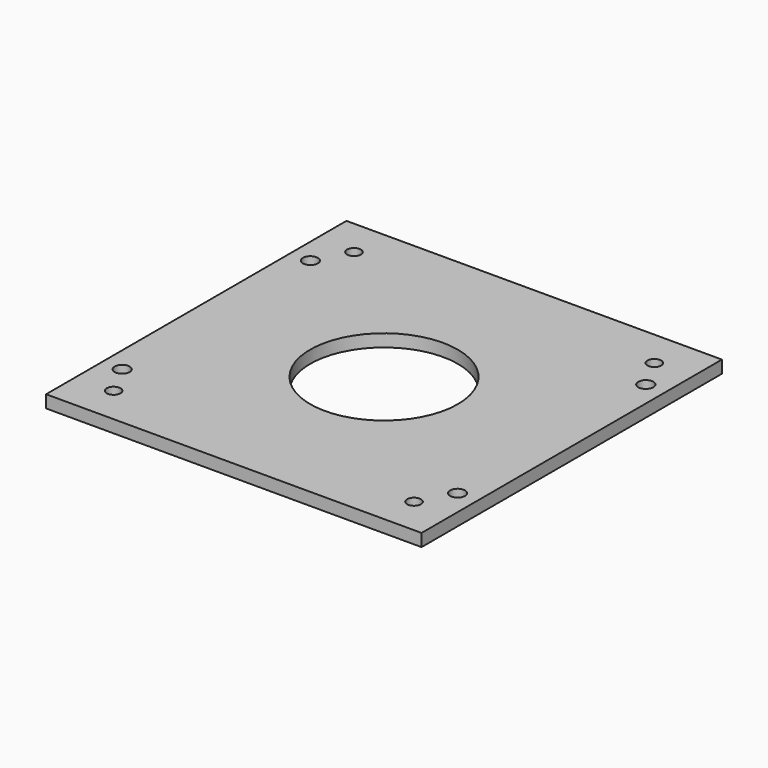
from build123d import *

# Parameters (mm, degrees)
F2_W            = 150
F2_H            = 150
F2_R            = 29.5
F3_DEPTH        = 5
F5_D            = 5.5
F5_COPIES_COUNT = 4
F6_R            = 3
F7_DEPTH        = 5.001


# Not quite as in the source:
# - a pattern or mirror of a feature is missing from the dataset's text; its kind, count and spacing are read off the source's solid
# - a feature names something its author has since deleted; it is built from what else it names


with BuildPart() as f3:
    # F2 (on Top) → F3 (new body)
    with BuildSketch(Plane.XY):
        Rectangle(F2_W, F2_H)
        Circle(F2_R, mode=Mode.SUBTRACT)
    extrude(amount=-F3_DEPTH)

    # F5 (through all)
    with Locations(Plane.XY):
        with Locations((-60, -60)):
            f5 = Hole(F5_D / 2)

    # F5_copies: F5 ×4 about axis
    f5_copies_axis = Axis((0, 0, 0), (0, 0, 1))
    for i in range(1, F5_COPIES_COUNT):
        add(f5.rotate(f5_copies_axis, i * 360 / F5_COPIES_COUNT), mode=Mode.SUBTRACT)

    # F6 (on Top) → F7 (cut, through all)
    with BuildSketch(Plane.XY):
        with Locations((-67, -47)):
            Circle(F6_R)
    f7 = extrude(amount=-F7_DEPTH, mode=Mode.SUBTRACT)

    # F7_copies: F7 across plane
    add(f7.mirror(Plane(origin=(0, 0, 0), x_dir=(0, 0, 1), z_dir=(1, 0, 0))), mode=Mode.SUBTRACT)

    # F7_copies1: F7 across plane
    add(f7.mirror(Plane.ZX), mode=Mode.SUBTRACT)

    # F7_copies2: F7 across plane
    add(f7.mirror(Plane(origin=(0, 0, 0), x_dir=(-0.5742821086, 0.818657474, 0), z_dir=(0.818657474, 0.5742821086, 0))), mode=Mode.SUBTRACT)


solid = f3.part
